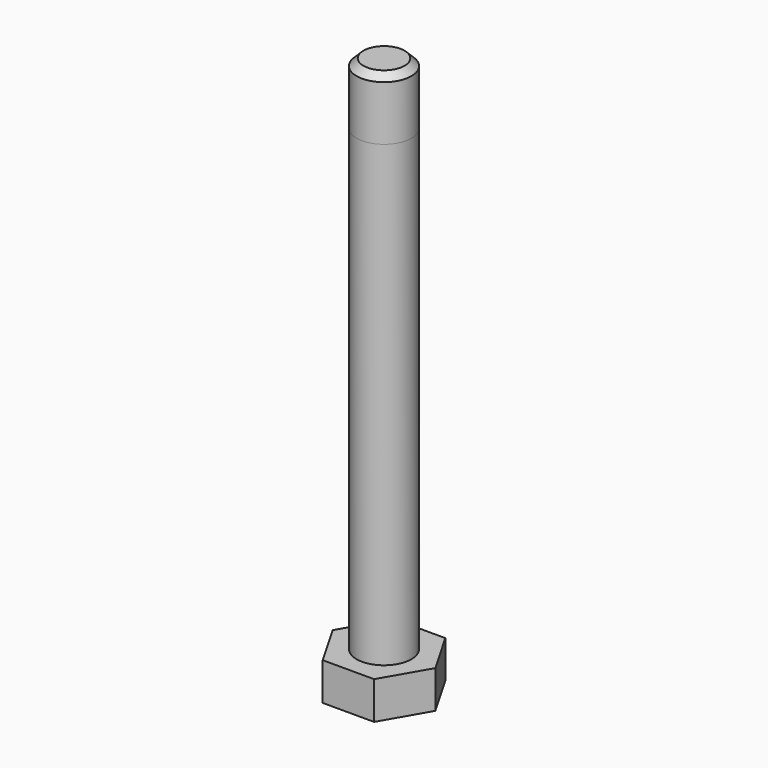
from build123d import *

# Parameters (mm, degrees)
F0_R      = 4
F1_DEPTH  = 5.5
F2_DEPTH  = 76
F3_DEPTH  = 5.5
F4_DEPTH  = 68
F5_SIZE   = 1
F5_2_SIZE = 1


with BuildPart() as f1:
    # F0 (on Top) → F1 (new body)
    with BuildSketch(Plane.XY):
        Polygon((3.7527767497, 6.5), (-3.7527767497, 6.5), (-7.5055534995, 0), (-3.7527767497, -6.5), (3.7527767497, -6.5), (7.5055534995, 0), align=None)
        Circle(F0_R, mode=Mode.SUBTRACT)
        Circle(F0_R)
    extrude(amount=-F1_DEPTH)

    # F0 (on Top) → F2 (join)
    with BuildSketch(Plane.XY):
        Circle(F0_R)
    extrude(amount=F2_DEPTH)

    # F5
    f5_edges = [f1.edges().sort_by_distance(p)[0] for p in [
        (-4, 0, 76),
    ]]
    chamfer(f5_edges, length=F5_SIZE)


with BuildPart() as f3:
    # F0 (on Top) → F3 (new body)
    with BuildSketch(Plane.XY):
        Polygon((3.7527767497, 6.5), (-3.7527767497, 6.5), (-7.5055534995, 0), (-3.7527767497, -6.5), (3.7527767497, -6.5), (7.5055534995, 0), align=None)
        Circle(F0_R, mode=Mode.SUBTRACT)
        Circle(F0_R)
    extrude(amount=-F3_DEPTH)

    # F0 (on Top) → F4 (join)
    with BuildSketch(Plane.XY):
        Circle(F0_R)
    extrude(amount=F4_DEPTH)

    # F5#2
    f5_2_edges = [f3.edges().sort_by_distance(p)[0] for p in [
        (-4, 0, 68),
    ]]
    chamfer(f5_2_edges, length=F5_2_SIZE)


solid = Compound([f1.part, f3.part])
